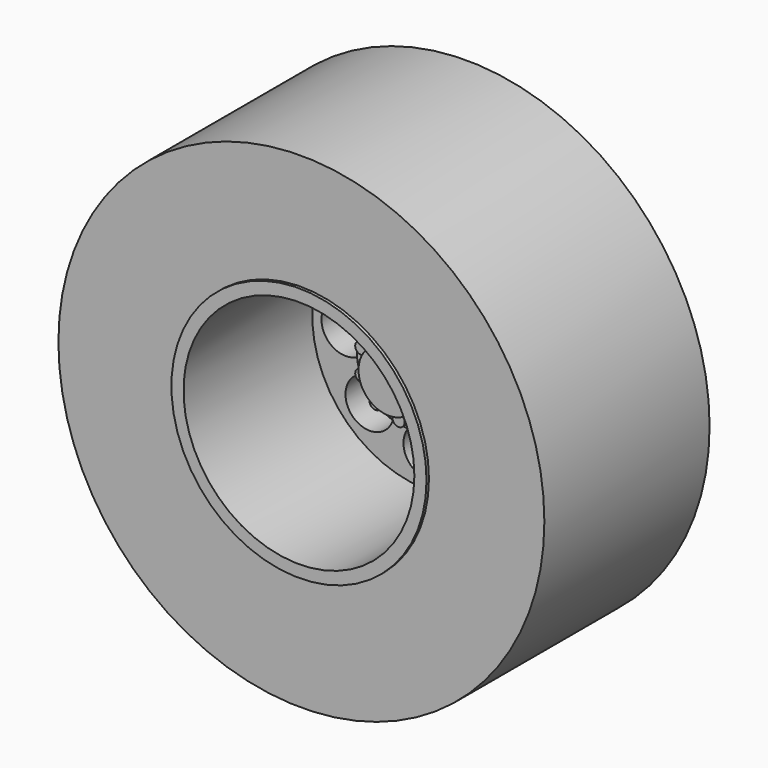
from build123d import *

# Parameters (mm, degrees)
F0_R      = 20
F1_DEPTH  = 17
F2_R      = 9.5
F3_DEPTH  = 13
F2_R_2    = 10.5
F4_DEPTH  = 0.25
F5_R      = 2
F6_DEPTH  = 25
F7_R      = 4.25
F8_DEPTH  = 2
F9_R      = 2.5
F10_DEPTH = 2
F11_R     = 0.5
F12_DEPTH = 1


# Not quite as in the source:
# - a feature names something its author has since deleted; it is built from what else it names


with BuildPart() as f1:
    # F0 (on Front) → F1 (new body)
    with BuildSketch(Plane.XZ):
        Circle(F0_R)
    extrude(amount=F1_DEPTH)

    # F2 (on face) → F3 (cut)
    with BuildSketch(Plane.XZ.offset(17)):
        Circle(F2_R)
    extrude(amount=-F3_DEPTH, mode=Mode.SUBTRACT)

    # F2 (on face) → F4 (join)
    with BuildSketch(Plane.XZ.offset(17)):
        Circle(F2_R_2)
        Circle(F2_R, mode=Mode.SUBTRACT)
    extrude(amount=F4_DEPTH)

    # F5 (on face) → F6 (cut)
    with BuildSketch(Plane.XZ.offset(4)):
        with Locations((0, 6.7485035397)):
            Circle(F5_R)
        with Locations((4.7719126158, 4.7719126158)):
            Circle(F5_R)
        with Locations((6.7485035397, 0)):
            Circle(F5_R)
        with Locations((4.7719126158, -4.7719126158)):
            Circle(F5_R)
        with Locations((0, -6.7485035397)):
            Circle(F5_R)
        with Locations((-4.7719126158, -4.7719126158)):
            Circle(F5_R)
        with Locations((-6.7485035397, 0)):
            Circle(F5_R)
        with Locations((-4.7719126158, 4.7719126158)):
            Circle(F5_R)
    extrude(amount=-F6_DEPTH, mode=Mode.SUBTRACT)

    # F7 (on face) → F8 (join)
    with BuildSketch(Plane.XZ.offset(4)):
        Circle(F7_R)
    extrude(amount=F8_DEPTH)

    # F9 (on face) → F10 (join)
    with BuildSketch(Plane.XZ.offset(6)):
        Circle(F9_R)
    extrude(amount=F10_DEPTH)

    # F11 (on face) → F12 (join)
    with BuildSketch(Plane.XZ.offset(6)):
        with Locations((0, 3.2268003561)):
            Circle(F11_R)
        with Locations((1.8966656614, 2.6105363255)):
            Circle(F11_R)
        with Locations((3.0688695054, -0.9971361475)):
            Circle(F11_R)
        with Locations((3.0688695054, 0.9971361475)):
            Circle(F11_R)
        with Locations((1.8966656614, -2.6105363255)):
            Circle(F11_R)
        with Locations((0, -3.2268003561)):
            Circle(F11_R)
        with Locations((-1.8966656614, -2.6105363255)):
            Circle(F11_R)
        with Locations((-3.0688695054, -0.9971361475)):
            Circle(F11_R)
        with Locations((-3.0688695054, 0.9971361475)):
            Circle(F11_R)
        with Locations((-1.8966656614, 2.6105363255)):
            Circle(F11_R)
    extrude(amount=F12_DEPTH)


solid = f1.part
